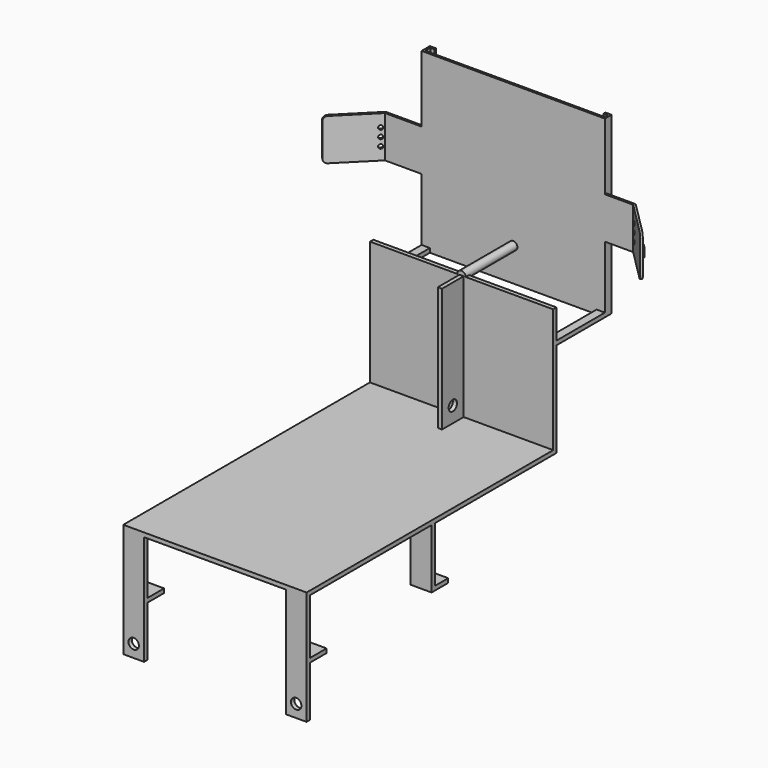
from build123d import *

# Parameters (mm, degrees)
F0_W      = 9
F0_H      = 10
F0_W_2    = 44
F0_H_2    = 16
F0_W_3    = 7
F0_R      = 1
F1_DEPTH  = 0.5
F3_R      = 0.5
F3_W      = 0.3535533906
F3_H      = 10
F4_DEPTH  = 0.5
F6_R      = 0.5
F6_W      = 0.3535533906
F6_H      = 10
F7_DEPTH  = 0.5
F8_R      = 1.25
F9_DEPTH  = 0.5
F10_R     = 1.25
F11_DEPTH = 0.5
F12_DEPTH = 0.5
F14_DEPTH = 15
F13_W     = 2
F13_H     = 14.5
F15_DEPTH = 1
F16_W     = 2
F16_H     = 1
F17_DEPTH = 1
F18_W     = 1
F18_H     = 29.75
F19_DEPTH = 6.5
F21_D     = 2.5
F21_DEPTH = 8
F21_TIP   = 0.7510757738
F23_DEPTH = 1
F25_DEPTH = 1
F26_R     = 1.25
F27_DEPTH = 1
F28_W     = 5
F28_H     = 1
F29_DEPTH = 5
F30_DEPTH = 14.25
F31_W     = 5
F31_H     = 4
F31_H_2   = 1
F32_DEPTH = 1
F34_DEPTH = 0.5
F35_W     = 1
F35_H     = 42
F36_DEPTH = 0.5
F38_DEPTH = 0.5
F39_W     = 0.5
F39_H     = 42
F39_W_2   = 1
F40_DEPTH = 0.5


# Not quite as in the source:
# - a feature of the source that left no trace in its solid (it failed there, or was rolled back) is left out
# - a feature names something its author has since deleted; it is built from what else it names


with BuildPart() as f1:
    # F0 (on Front) → F1 (new body)
    with BuildSketch(Plane.XZ):
        with Locations((-25.5, 0)):
            Rectangle(F0_W, F0_H)
        with Locations((1, 13)):
            Rectangle(F0_W_2, F0_H_2)
        with Locations((1, 0)):
            Rectangle(F0_W_2, F0_H)
        with Locations((26.5, 0)):
            Rectangle(F0_W_3, F0_H)
        with Locations((1, -13)):
            Rectangle(F0_W_2, F0_H_2)
        with Locations((1, -13)):
            Circle(F0_R, mode=Mode.SUBTRACT)
    extrude(amount=F1_DEPTH)

    # F3 (on face) → F4 (join)
    with BuildSketch(Plane(origin=(15, 15, 0), x_dir=(0.7071067812, -0.7071067812, 0), z_dir=(-0.7071067812, -0.7071067812, 0))):
        with BuildLine():
            Line((21.5667568262, 5), (21.5667568262, -5))
            Line((21.5667568262, -5), (32.2132034356, -5))
            ThreePointArc((32.2132034356, -5), (32.9203102168, -4.7071067812), (33.2132034356, -4))
            Line((33.2132034356, -4), (33.2132034356, 4))
            ThreePointArc((33.2132034356, 4), (32.9203102168, 4.7071067812), (32.2132034356, 5))
            Line((32.2132034356, 5), (21.5667568262, 5))
        make_face()
        with Locations((23.2132034356, -2)):
            Circle(F3_R, mode=Mode.SUBTRACT)
        with Locations((23.2132034356, 0)):
            Circle(F3_R, mode=Mode.SUBTRACT)
        with Locations((23.2132034356, 2)):
            Circle(F3_R, mode=Mode.SUBTRACT)
        with Locations((21.3899801309, 0)):
            Rectangle(F3_W, F3_H)
    extrude(amount=F4_DEPTH)

    # F6 (on face) → F7 (join)
    with BuildSketch(Plane(origin=(-15, 15, 0), x_dir=(0.7071067812, 0.7071067812, 0), z_dir=(0.7071067812, -0.7071067812, 0))):
        with BuildLine():
            Line((-21.5667568262, -5), (-21.5667568262, 5))
            Line((-21.5667568262, 5), (-32.2132034356, 5))
            ThreePointArc((-32.2132034356, 5), (-32.9203102168, 4.7071067812), (-33.2132034356, 4))
            Line((-33.2132034356, 4), (-33.2132034356, -4))
            ThreePointArc((-33.2132034356, -4), (-32.9203102168, -4.7071067812), (-32.2132034356, -5))
            Line((-32.2132034356, -5), (-21.5667568262, -5))
        make_face()
        with Locations((-22.2132034356, -2)):
            Circle(F6_R, mode=Mode.SUBTRACT)
        with Locations((-22.2132034356, 0)):
            Circle(F6_R, mode=Mode.SUBTRACT)
        with Locations((-22.2132034356, 2)):
            Circle(F6_R, mode=Mode.SUBTRACT)
        with Locations((-21.3899801309, 0)):
            Rectangle(F6_W, F6_H)
    extrude(amount=F7_DEPTH)

    # F8 (on face) → F9 (join)
    with BuildSketch(Plane(origin=(15, 15, 0), x_dir=(-0.7071067812, 0.7071067812, 0), z_dir=(0.7071067812, 0.7071067812, 0))):
        with Locations((-30.7632034356, 0)):
            Circle(F8_R)
    extrude(amount=F9_DEPTH)

    # F10 (on face) → F11 (join)
    with BuildSketch(Plane(origin=(-15, 15, 0), x_dir=(-0.7071067812, -0.7071067812, 0), z_dir=(-0.7071067812, 0.7071067812, 0))):
        with Locations((30.7632034356, 0)):
            Circle(F10_R)
    extrude(amount=F11_DEPTH)

    # F0 (on Front) → F12 (join)
    with BuildSketch(Plane.XZ):
        with Locations((1, 13)):
            Rectangle(F0_W_2, F0_H_2)
        with Locations((1, -13)):
            Rectangle(F0_W_2, F0_H_2)
        with Locations((1, -13)):
            Circle(F0_R, mode=Mode.SUBTRACT)
    extrude(amount=F12_DEPTH)

    # F0 (on Front) → F14 (join)
    with BuildSketch(Plane.XZ):
        with Locations((1, -13)):
            Circle(F0_R)
    extrude(amount=F14_DEPTH)

    # F13 (on face) → F15 (join)
    with BuildSketch(Plane(origin=(0, 0, -21), x_dir=(1, 0, 0), z_dir=(0, 0, -1))):
        with Locations((-20, 7.75)):
            Rectangle(F13_W, F13_H)
        with Locations((22, 7.75)):
            Rectangle(F13_W, F13_H)
    extrude(amount=-F15_DEPTH)

    # F16 (on face) → F17 (join)
    with BuildSketch(Plane.XZ.offset(15)):
        with BuildLine():
            Line((-19, -21), (-21, -21))
            Line((-21, -21), (-21, -42.75))
            Line((-21, -42.75), (23, -42.75))
            Line((23, -42.75), (23, -21))
            Line((23, -21), (21, -21))
            Line((21, -21), (21, -20))
            Line((21, -20), (23, -20))
            Line((23, -20), (23, -13))
            Line((23, -13), (2, -13))
            ThreePointArc((2, -13), (1, -14), (0, -13))
            Line((0, -13), (-21, -13))
            Line((-21, -13), (-21, -20))
            Line((-21, -20), (-19, -20))
            Line((-19, -20), (-19, -21))
        make_face()
        with Locations((-20, -20.5)):
            Rectangle(F16_W, F16_H)
        with BuildLine():
            ThreePointArc((2, -13), (1, -12), (0, -13))
            Line((0, -13), (2, -13))
        make_face()
        with BuildLine():
            Line((2, -13), (0, -13))
            ThreePointArc((0, -13), (1, -14), (2, -13))
        make_face()
        with Locations((22, -20.5)):
            Rectangle(F16_W, F16_H)
    extrude(amount=F17_DEPTH)

    # F18 (on face) → F19 (join)
    with BuildSketch(Plane.XZ.offset(16)):
        with Locations((1, -27.875)):
            Rectangle(F18_W, F18_H)
    extrude(amount=F19_DEPTH)

    # F21
    with Locations(Plane.YZ.offset(1.5)):
        with Locations((-19.25, -39)):
            Hole(F21_D / 2, depth=F21_DEPTH)
            with Locations((0, 0, -(F21_DEPTH + F21_TIP / 2))):  # 118° drill point
                Cone(0, F21_D / 2, F21_TIP, mode=Mode.SUBTRACT)

    # F22 (on face) → F23 (join)
    with BuildSketch(Plane(origin=(0, 0, -42.75), x_dir=(1, 0, 0), z_dir=(0, 0, -1))):
        Polygon((-21, 15), (23, 15), (23, 16), (1.5, 16), (1.5, 22.5), (0.5, 22.5), (0.5, 16), (-21, 16), align=None)
    extrude(amount=F23_DEPTH)

    # F22 (on face) → F25 (join)
    with BuildSketch(Plane(origin=(0, 0, -42.75), x_dir=(1, 0, 0), z_dir=(0, 0, -1))):
        Polygon((1.5, 16), (23, 16), (23, 51.5), (18, 51.5), (18, 52.5), (23, 52.5), (23, 53), (23, 90), (-21, 90), (-21, 52.5), (-16, 52.5), (-16, 51.5), (-21, 51.5), (-21, 16), (0.5, 16), (0.5, 22.5), (1.5, 22.5), align=None)
        Polygon((-21, 15), (23, 15), (23, 16), (1.5, 16), (1.5, 22.5), (0.5, 22.5), (0.5, 16), (-21, 16), align=None)
    extrude(amount=F25_DEPTH)

    # F26 (on face) → F27 (join)
    with BuildSketch(Plane.XZ.offset(90)):
        Polygon((-16, -43.75), (-21, -43.75), (-21, -58), (-21, -70.1), (-16, -70.1), align=None)
        with Locations((-18.5, -67.075)):
            Circle(F26_R, mode=Mode.SUBTRACT)
        Polygon((23, -43.75), (18, -43.75), (18, -70.1), (23, -70.1), (23, -58), align=None)
        with Locations((20.5, -67.075)):
            Circle(F26_R, mode=Mode.SUBTRACT)
    extrude(amount=-F27_DEPTH)

    # F28 (on face) → F29 (join)
    with BuildSketch(Plane(origin=(0, -89, 0), x_dir=(-1, 0, 0), z_dir=(0, 1, 0))):
        with Locations((18.5, -57.5)):
            Rectangle(F28_W, F28_H)
        with Locations((-20.5, -57.5)):
            Rectangle(F28_W, F28_H)
    extrude(amount=F29_DEPTH)

    # F22 (on face) → F30 (join)
    with BuildSketch(Plane(origin=(0, 0, -42.75), x_dir=(1, 0, 0), z_dir=(0, 0, -1))):
        Polygon((-21, 52), (-21, 51.5), (-16, 51.5), (-16, 52.5), (-21, 52.5), align=None)
        Polygon((18, 51.5), (23, 51.5), (23, 52), (23, 52.5), (18, 52.5), align=None)
    extrude(amount=F30_DEPTH)

    # F31 (on face) → F32 (join)
    with BuildSketch(Plane(origin=(0, 0, -57), x_dir=(1, 0, 0), z_dir=(0, 0, -1))):
        with Locations((20.5, 49.5)):
            Rectangle(F31_W, F31_H)
        with Locations((20.5, 52)):
            Rectangle(F31_W, F31_H_2)
        with Locations((-18.5, 49.5)):
            Rectangle(F31_W, F31_H)
        with Locations((-18.5, 52)):
            Rectangle(F31_W, F31_H_2)
    extrude(amount=F32_DEPTH)

    # F33 (on face) → F34 (join)
    with BuildSketch(Plane.YZ.offset(23)):
        Polygon((0, 21), (0, 5), (0, -5), (0, -21), (1.5, -21), (1.5, 21), align=None)
    extrude(amount=-F34_DEPTH)

    # F35 (on face) → F36 (join)
    with BuildSketch(Plane(origin=(0, 1.5, 0), x_dir=(-1, 0, 0), z_dir=(0, 1, 0))):
        with Locations((-22, 0)):
            Rectangle(F35_W, F35_H)
    extrude(amount=-F36_DEPTH)

    # F37 (on face) → F38 (join)
    with BuildSketch(Plane(origin=(-21, 0, 0), x_dir=(0, -1, 0), z_dir=(-1, 0, 0))):
        Polygon((-1.5, -21), (0, -21), (0, -5), (0, 21), (-1.5, 21), align=None)
    extrude(amount=-F38_DEPTH)

    # F39 (on face) → F40 (join)
    with BuildSketch(Plane(origin=(0, 1.5, 0), x_dir=(-1, 0, 0), z_dir=(0, 1, 0))):
        with Locations((20.75, 0)):
            Rectangle(F39_W, F39_H)
        with Locations((20, 0)):
            Rectangle(F39_W_2, F39_H)
    extrude(amount=F40_DEPTH)


solid = f1.part
